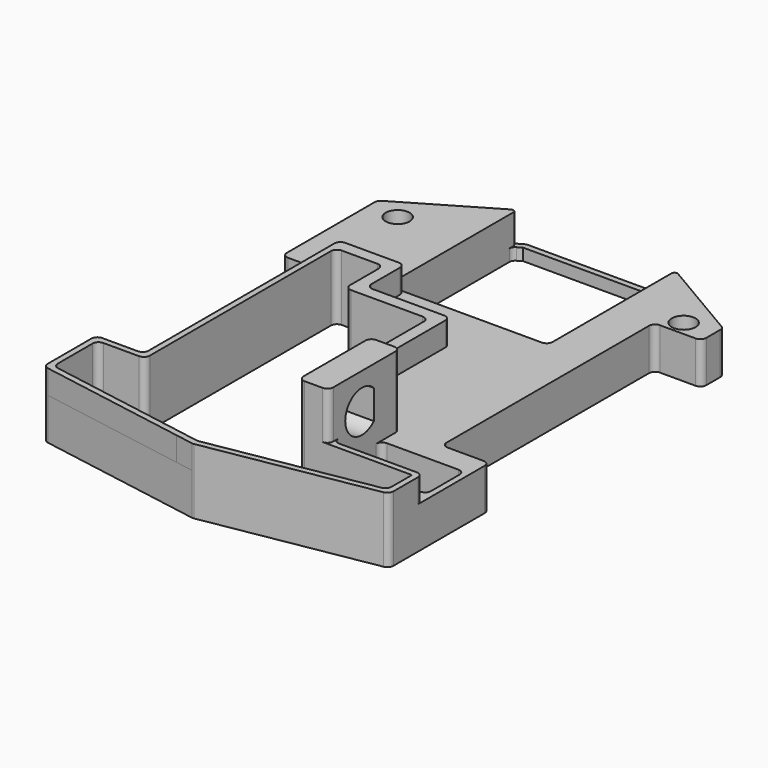
from build123d import *

# Parameters (mm, degrees)
F1_W          = 1
F1_H          = 1
F1_R          = 2
F2_DEPTH      = 7
F4_DEPTH      = 4
F6_DEPTH      = 8
F8_DEPTH      = 25
F9_W          = 1
F9_H          = 39
F10_DEPTH     = 4
F11_DEPTH     = 2
F12_T1_DEPTH  = 7
F12_T3_DEPTH  = 6.5
F12_T5_DEPTH  = 11
F12_T7_DEPTH  = 2
F12_T9_DEPTH  = 9.8597039194
F12_T11_DEPTH = 6.5
F12_T13_DEPTH = 12
F12_T15_DEPTH = 15.2116961582
F12_T17_DEPTH = 10.5
F12_T19_DEPTH = 11.8620773197
F12_T21_DEPTH = 6.5
F12_T23_DEPTH = 3.3615627907
F12_T25_DEPTH = 16
F12_T27_DEPTH = 14.5
F12_T29_DEPTH = 10.5
F12_T31_DEPTH = 24
F13_R         = 0.5


# Not quite as in the source:
# - a fillet or chamfer that OpenCascade refuses, or shapes differently, is made with other operations: its cross-section is extruded or revolved along the edge and cut away or added


with BuildPart() as f2:
    # F1 (on Top) → F2 (new body)
    with BuildSketch(Plane.XY):
        with Locations((-28.5, 11.5000484542)):
            Rectangle(F1_W, F1_H)
        Polygon((-21, 12.0000484542), (-28, 12.0000484542), (-28, 11.0000484542), (-20, 11.0000484542), (-20, 51.0000484542), (-21, 51.0000484542), align=None)
        with BuildLine():
            Line((29, 66.5), (29, 71.0000484542))
            Line((29, 71.0000484542), (14, 79.8237382314))
            Line((14, 79.8237382314), (14, 78.6635514624))
            Line((14, 78.6635514624), (14, 53.0002302017))
            Line((14, 53.0002302017), (-13, 53.0002302017))
            Line((-13, 53.0002302017), (-13, 79.2517974475))
            Line((-13, 79.2517974475), (-13, 80.4119842166))
            Line((-13, 80.4119842166), (-29, 71.0000484542))
            Line((-29, 71.0000484542), (-29, 12.0000484542))
            Line((-29, 12.0000484542), (-28, 12.0000484542))
            Line((-28, 12.0000484542), (-28, 51.0000484542))
            Line((-28, 51.0000484542), (-21, 51.0000484542))
            Line((-21, 51.0000484542), (-20, 51.0000484542))
            Line((-20, 51.0000484542), (-12, 51.0000484542))
            Line((-12, 51.0000484542), (-12, 43.0000484542))
            Line((-12, 43.0000484542), (2, 43.0000484542))
            Line((2, 43.0000484542), (2, 18))
            Line((2, 18), (9, 18))
            Line((9, 18), (14, 18))
            Line((14, 18), (28, 18))
            Line((28, 18), (28, 10.0000484542))
            Line((28, 10.0000484542), (28, 7.0000484542))
            Line((28, 7.0000484542), (28, 1.8423876859))
            Line((28, 1.8423876859), (3, -2.4679989126))
            Line((3, -2.4679989126), (3, 0))
            ThreePointArc((3, 0), (0, 3), (-3, 0))
            Line((-3, 0), (-3, -2.4679989126))
            Line((-3, -2.4679989126), (-28, 1.8423876859))
            Line((-28, 1.8423876859), (-28, 11.0000484542))
            Line((-28, 11.0000484542), (-29, 11.0000484542))
            Line((-29, 11.0000484542), (-29, 1.0000484542))
            Line((-29, 1.0000484542), (0, -4))
            Line((0, -4), (29, 1.0000484542))
            Line((29, 1.0000484542), (29, 22))
            Line((29, 22), (21, 22))
            Line((21, 22), (21, 66.5))
            Line((21, 66.5), (29, 66.5))
        make_face()
        Circle(F1_R, mode=Mode.SUBTRACT)
        with Locations((-24, 69)):
            Circle(F1_R, mode=Mode.SUBTRACT)
        with Locations((24, 69)):
            Circle(F1_R, mode=Mode.SUBTRACT)
        Polygon((9, 7.0000484542), (28, 7.0000484542), (28, 10.0000484542), (14, 10.0000484542), (14, 18), (9, 18), align=None)
    extrude(amount=F2_DEPTH)

    # F3 (on face) → F4 (join)
    with BuildSketch(Plane.XY.offset(7)):
        Polygon((4, 22), (4, 33), (4, 45.0000484542), (-10, 45.0000484542), (-10, 53.0000484542), (-21, 53.0000484542), (-21, 51.0000484542), (-21, 12.0000484542), (-28, 12.0000484542), (-29, 12.0000484542), (-29, 1.0000484542), (-3.1699085155, -3.4534587527), (0, -4), (29, 1.0000484542), (29, 8.0000484542), (14, 8.0000484542), (14, 10.0000484542), (14, 18), (14, 20), (14, 22), align=None)
        Polygon((0, -2.9852453044), (-3, -2.4679989126), (-28, 1.8423876859), (-28, 11.0000484542), (-20, 11.0000484542), (-20, 51.0000484542), (-12, 51.0000484542), (-12, 43.0000484542), (2, 43.0000484542), (2, 33), (2, 31), (2, 20), (9, 20), (9, 18), (9, 7.0000484542), (28, 7.0000484542), (28, 1.8423876859), (3, -2.4679989126), align=None, mode=Mode.SUBTRACT)
    extrude(amount=F4_DEPTH)

    # F5 (on face) → F6 (join)
    with BuildSketch(Plane.XY.offset(11)):
        Polygon((9, 20), (9, 7.0000484542), (14, 7.0000484542), (14, 8.0000484542), (14, 22), (9, 22), align=None)
    extrude(amount=F6_DEPTH)

    # F7 (on face) → F8 (cut)
    with BuildSketch(Plane.YZ.offset(29)):
        with BuildLine():
            Line((16.5000484542, 10.5505102572), (16.5000484542, 15.4494897428))
            ThreePointArc((16.5000484542, 15.4494897428), (10.5000484542, 13), (16.5000484542, 10.5505102572))
        make_face()
    extrude(amount=-F8_DEPTH, mode=Mode.SUBTRACT)

    # F9 (on face) → F10 (cut)
    with BuildSketch(Plane.XY.offset(7)):
        with Locations((-28.5, 31.5000484542)):
            Rectangle(F9_W, F9_H)
    extrude(amount=-F10_DEPTH, mode=Mode.SUBTRACT)

    # F1 (on Top) → F11 (join)
    with BuildSketch(Plane.XY):
        Polygon((14, 78.6635514624), (14, 79.8237382314), (12, 81.0002302017), (-12, 81.0002302017), (-13, 80.4119842166), (-13, 79.2517974475), (-11.7276874419, 80.0002302017), (11.7276874419, 80.0002302017), align=None)
    extrude(amount=F11_DEPTH)

    # F12: fillet of radius 1 on 48 edges, made by hand

    # F12_s2 → F12_t1 (join)
    with BuildSketch(Plane.XY):
        with BuildLine():
            ThreePointArc((-13, 54.0002302017), (-12.7071067812, 53.2931234205), (-12, 53.0002302017))
            Line((-12, 53.0002302017), (-13, 53.0002302017))
            Line((-13, 53.0002302017), (-13, 54.0002302017))
        make_face()
        with BuildLine():
            ThreePointArc((13, 53.0002302017), (13.7071067812, 53.2931234205), (14, 54.0002302017))
            Line((14, 54.0002302017), (14, 53.0002302017))
            Line((14, 53.0002302017), (13, 53.0002302017))
        make_face()
        with BuildLine():
            ThreePointArc((21, 23), (21.2928932188, 22.2928932188), (22, 22))
            Line((22, 22), (21, 22))
            Line((21, 22), (21, 23))
        make_face()
        with BuildLine():
            ThreePointArc((22, 66.5), (21.2928932188, 66.2071067812), (21, 65.5))
            Line((21, 65.5), (21, 66.5))
            Line((21, 66.5), (22, 66.5))
        make_face()
        with BuildLine():
            ThreePointArc((-22, 51.0000484542), (-21.2928932188, 50.7071552354), (-21, 50.0000484542))
            Line((-21, 50.0000484542), (-21, 51.0000484542))
            Line((-21, 51.0000484542), (-22, 51.0000484542))
        make_face()
        with BuildLine():
            ThreePointArc((14, 11.0000484542), (14.2928932188, 10.2929416731), (15, 10.0000484542))
            Line((15, 10.0000484542), (14, 10.0000484542))
            Line((14, 10.0000484542), (14, 11.0000484542))
        make_face()
        with BuildLine():
            ThreePointArc((14, 17), (14.2928932188, 17.7071067812), (15, 18))
            Line((15, 18), (14, 18))
            Line((14, 18), (14, 17))
        make_face()
        with BuildLine():
            ThreePointArc((28, 17), (27.7071067812, 17.7071067812), (27, 18))
            Line((27, 18), (28, 18))
            Line((28, 18), (28, 17))
        make_face()
        with BuildLine():
            ThreePointArc((9, 17), (8.7071067812, 17.7071067812), (8, 18))
            Line((8, 18), (9, 18))
            Line((9, 18), (9, 17))
        make_face()
        with BuildLine():
            ThreePointArc((27, 10.0000484542), (27.7071067812, 10.2929416731), (28, 11.0000484542))
            Line((28, 11.0000484542), (28, 10.0000484542))
            Line((28, 10.0000484542), (27, 10.0000484542))
        make_face()
        with BuildLine():
            ThreePointArc((-4.1699085155, -2.2662885931), (-3.3557595618, -2.0456517769), (-3, -1.2808287531))
            Line((-3, -1.2808287531), (-3, -2.4679989126))
            Line((-3, -2.4679989126), (-4.1699085155, -2.2662885931))
        make_face()
        with BuildLine():
            ThreePointArc((3, -1.2808287531), (3.3557595618, -2.0456517769), (4.1699085155, -2.2662885931))
            Line((4.1699085155, -2.2662885931), (3, -2.4679989126))
            Line((3, -2.4679989126), (3, -1.2808287531))
        make_face()
    extrude(amount=F12_T1_DEPTH)

    # F12_s4 → F12_t3 (join)
    with BuildSketch(Plane.XY.offset(4.5)):
        with BuildLine():
            ThreePointArc((-9, 45.0000484542), (-9.7071067812, 45.2929416731), (-10, 46.0000484542))
            Line((-10, 46.0000484542), (-10, 45.0000484542))
            Line((-10, 45.0000484542), (-9, 45.0000484542))
        make_face()
        with BuildLine():
            ThreePointArc((5, 22), (4.2928932188, 22.2928932188), (4, 23))
            Line((4, 23), (4, 22))
            Line((4, 22), (5, 22))
        make_face()
        with BuildLine():
            ThreePointArc((15, 8.0000484542), (14.2928932188, 8.2929416731), (14, 9.0000484542))
            Line((14, 9.0000484542), (14, 8.0000484542))
            Line((14, 8.0000484542), (15, 8.0000484542))
        make_face()
        with BuildLine():
            ThreePointArc((9, 19), (8.7071067812, 19.7071067812), (8, 20))
            Line((8, 20), (9, 20))
            Line((9, 20), (9, 19))
        make_face()
    extrude(amount=F12_T3_DEPTH)

    # F12_s6 → F12_t5 (join)
    with BuildSketch(Plane.XY):
        with BuildLine():
            ThreePointArc((-22, 12.0000484542), (-21.2928932188, 12.2929416731), (-21, 13.0000484542))
            Line((-21, 13.0000484542), (-21, 12.0000484542))
            Line((-21, 12.0000484542), (-22, 12.0000484542))
        make_face()
        with BuildLine():
            ThreePointArc((2, 42.0000484542), (1.7071067812, 42.7071552354), (1, 43.0000484542))
            Line((1, 43.0000484542), (2, 43.0000484542))
            Line((2, 43.0000484542), (2, 42.0000484542))
        make_face()
        with BuildLine():
            ThreePointArc((-12, 50.0000484542), (-12.2928932188, 50.7071552354), (-13, 51.0000484542))
            Line((-13, 51.0000484542), (-12, 51.0000484542))
            Line((-12, 51.0000484542), (-12, 50.0000484542))
        make_face()
        with BuildLine():
            ThreePointArc((-19, 51.0000484542), (-19.7071067812, 50.7071552354), (-20, 50.0000484542))
            Line((-20, 50.0000484542), (-20, 51.0000484542))
            Line((-20, 51.0000484542), (-19, 51.0000484542))
        make_face()
        with BuildLine():
            ThreePointArc((-28, 10.0000484542), (-27.7071067812, 10.7071552354), (-27, 11.0000484542))
            Line((-27, 11.0000484542), (-28, 11.0000484542))
            Line((-28, 11.0000484542), (-28, 10.0000484542))
        make_face()
        with BuildLine():
            ThreePointArc((-28, 2.6847269175), (-27.7648230238, 2.0404864793), (-27.1699085155, 1.6992670775))
            Line((-27.1699085155, 1.6992670775), (-28, 1.8423876859))
            Line((-28, 1.8423876859), (-28, 2.6847269175))
        make_face()
        with BuildLine():
            ThreePointArc((27.1699085155, 1.6992670775), (27.7648230238, 2.0404864793), (28, 2.6847269175))
            Line((28, 2.6847269175), (28, 1.8423876859))
            Line((28, 1.8423876859), (27.1699085155, 1.6992670775))
        make_face()
    extrude(amount=F12_T5_DEPTH)

    # F12_s8 → F12_t7 (join)
    with BuildSketch(Plane.XY):
        with BuildLine():
            ThreePointArc((-12.5070269726, 79.5417868517), (-12.8680515459, 79.1763307452), (-13, 78.6798566636))
            Line((-13, 78.6798566636), (-13, 79.2517974475))
            Line((-13, 79.2517974475), (-12.5070269726, 79.5417868517))
        make_face()
        with BuildLine():
            ThreePointArc((13.5070269726, 78.9535408665), (13.8680515459, 78.5880847601), (14, 78.0916106785))
            Line((14, 78.0916106785), (14, 78.6635514624))
            Line((14, 78.6635514624), (13.5070269726, 78.9535408665))
        make_face()
    extrude(amount=F12_T7_DEPTH)

    # F12_s10 → F12_t9 (cut)
    with BuildSketch(Plane.XY.offset(-1.4298519597)):
        with BuildLine():
            ThreePointArc((28.5070269726, 71.2900378584), (28.8680515459, 70.924581752), (29, 70.4281076704))
            Line((29, 70.4281076704), (29, 71.0000484542))
            Line((29, 71.0000484542), (28.5070269726, 71.2900378584))
        make_face()
        with BuildLine():
            ThreePointArc((-28.5070269726, 71.2900378584), (-28.8680515459, 70.924581752), (-29, 70.4281076704))
            Line((-29, 70.4281076704), (-29, 71.0000484542))
            Line((-29, 71.0000484542), (-28.5070269726, 71.2900378584))
        make_face()
    extrude(amount=F12_T9_DEPTH, mode=Mode.SUBTRACT)

    # F12_s12 → F12_t11 (cut)
    with BuildSketch(Plane.XY.offset(7)):
        with BuildLine():
            ThreePointArc((4, 44.0000484542), (3.7071067812, 44.7071552354), (3, 45.0000484542))
            Line((3, 45.0000484542), (4, 45.0000484542))
            Line((4, 45.0000484542), (4, 44.0000484542))
        make_face()
        with BuildLine():
            ThreePointArc((-10, 52.0000484542), (-10.2928932188, 52.7071552354), (-11, 53.0000484542))
            Line((-11, 53.0000484542), (-10, 53.0000484542))
            Line((-10, 53.0000484542), (-10, 52.0000484542))
        make_face()
        with BuildLine():
            ThreePointArc((-20, 53.0000484542), (-20.7071067812, 52.7071552354), (-21, 52.0000484542))
            Line((-21, 52.0000484542), (-21, 53.0000484542))
            Line((-21, 53.0000484542), (-20, 53.0000484542))
        make_face()
        with BuildLine():
            ThreePointArc((3, 20), (2.2928932188, 20.2928932188), (2, 21))
            Line((2, 21), (2, 20))
            Line((2, 20), (3, 20))
        make_face()
        with BuildLine():
            ThreePointArc((28, 8.0000484542), (28.7071067812, 7.7071552354), (29, 7.0000484542))
            Line((29, 7.0000484542), (29, 8.0000484542))
            Line((29, 8.0000484542), (28, 8.0000484542))
        make_face()
    extrude(amount=F12_T11_DEPTH, mode=Mode.SUBTRACT)

    # F12_s14 → F12_t13 (cut)
    with BuildSketch(Plane.XY.offset(-2.5)):
        with BuildLine():
            ThreePointArc((28, 22), (28.7071067812, 21.7071067812), (29, 21))
            Line((29, 21), (29, 22))
            Line((29, 22), (28, 22))
        make_face()
        with BuildLine():
            ThreePointArc((29, 67.5), (28.7071067812, 66.7928932188), (28, 66.5))
            Line((28, 66.5), (29, 66.5))
            Line((29, 66.5), (29, 67.5))
        make_face()
        with BuildLine():
            ThreePointArc((3, 18), (2.2928932188, 18.2928932188), (2, 19))
            Line((2, 19), (2, 18))
            Line((2, 18), (3, 18))
        make_face()
    extrude(amount=F12_T13_DEPTH, mode=Mode.SUBTRACT)

    # F12_s16 → F12_t15 (cut)
    with BuildSketch(Plane.XY.offset(-2.1058480791)):
        with BuildLine():
            ThreePointArc((29, 1.8423876859), (28.7648230238, 1.1981472477), (28.1699085155, 0.8569278458))
            Line((28.1699085155, 0.8569278458), (29, 1.0000484542))
            Line((29, 1.0000484542), (29, 1.8423876859))
        make_face()
        with BuildLine():
            ThreePointArc((-28.1699085155, 0.8569278458), (-28.7648230238, 1.1981472477), (-29, 1.8423876859))
            Line((-29, 1.8423876859), (-29, 1.0000484542))
            Line((-29, 1.0000484542), (-28.1699085155, 0.8569278458))
        make_face()
    extrude(amount=F12_T15_DEPTH, mode=Mode.SUBTRACT)

    # F12_s18 → F12_t17 (cut)
    with BuildSketch(Plane.XY.offset(3)):
        with BuildLine():
            ThreePointArc((-28, 12.0000484542), (-28.7071067812, 11.7071552354), (-29, 11.0000484542))
            Line((-29, 11.0000484542), (-29, 12.0000484542))
            Line((-29, 12.0000484542), (-28, 12.0000484542))
        make_face()
    extrude(amount=F12_T17_DEPTH, mode=Mode.SUBTRACT)

    # F12_s20 → F12_t19 (cut)
    with BuildSketch(Plane.XY.offset(-0.4310386598)):
        with BuildLine():
            ThreePointArc((-0.1699085155, -3.9707051445), (0, -3.9852453044), (0.1699085155, -3.9707051445))
            Line((0.1699085155, -3.9707051445), (0, -4))
            Line((0, -4), (-0.1699085155, -3.9707051445))
        make_face()
    extrude(amount=F12_T19_DEPTH, mode=Mode.SUBTRACT)

    # F12_s22 → F12_t21 (cut)
    with BuildSketch(Plane.XY.offset(3)):
        with BuildLine():
            ThreePointArc((-28, 51.0000484542), (-28.7071067812, 51.2929416731), (-29, 52.0000484542))
            Line((-29, 52.0000484542), (-29, 51.0000484542))
            Line((-29, 51.0000484542), (-28, 51.0000484542))
        make_face()
    extrude(amount=F12_T21_DEPTH, mode=Mode.SUBTRACT)

    # F12_s24 → F12_t23 (cut)
    with BuildSketch(Plane.XY.offset(-0.6807813954)):
        with BuildLine():
            ThreePointArc((-12.2347144144, 80.8621603897), (-11.9904323866, 80.965095526), (-11.7276874419, 81.0002302017))
            Line((-11.7276874419, 81.0002302017), (-12, 81.0002302017))
            Line((-12, 81.0002302017), (-12.2347144144, 80.8621603897))
        make_face()
        with BuildLine():
            ThreePointArc((11.7276874419, 81.0002302017), (11.9904323866, 80.965095526), (12.2347144144, 80.8621603897))
            Line((12.2347144144, 80.8621603897), (12, 81.0002302017))
            Line((12, 81.0002302017), (11.7276874419, 81.0002302017))
        make_face()
    extrude(amount=F12_T23_DEPTH, mode=Mode.SUBTRACT)

    # F12_s26 → F12_t25 (cut)
    with BuildSketch(Plane.XY.offset(-2.5)):
        with BuildLine():
            ThreePointArc((-11, 43.0000484542), (-11.7071067812, 43.2929416731), (-12, 44.0000484542))
            Line((-12, 44.0000484542), (-12, 43.0000484542))
            Line((-12, 43.0000484542), (-11, 43.0000484542))
        make_face()
        with BuildLine():
            ThreePointArc((-20, 12.0000484542), (-20.2928932188, 11.2929416731), (-21, 11.0000484542))
            Line((-21, 11.0000484542), (-20, 11.0000484542))
            Line((-20, 11.0000484542), (-20, 12.0000484542))
        make_face()
    extrude(amount=F12_T25_DEPTH, mode=Mode.SUBTRACT)

    # F12_s28 → F12_t27 (cut)
    with BuildSketch(Plane.XY.offset(7)):
        with BuildLine():
            ThreePointArc((13, 22), (13.7071067812, 21.7071067812), (14, 21))
            Line((14, 21), (14, 22))
            Line((14, 22), (13, 22))
        make_face()
    extrude(amount=F12_T27_DEPTH, mode=Mode.SUBTRACT)

    # F12_s30 → F12_t29 (cut)
    with BuildSketch(Plane.XY.offset(11)):
        with BuildLine():
            ThreePointArc((10, 22), (9.2928932188, 21.7071067812), (9, 21))
            Line((9, 21), (9, 22))
            Line((9, 22), (10, 22))
        make_face()
        with BuildLine():
            ThreePointArc((14, 8.0000484542), (13.7071067812, 7.2929416731), (13, 7.0000484542))
            Line((13, 7.0000484542), (14, 7.0000484542))
            Line((14, 7.0000484542), (14, 8.0000484542))
        make_face()
    extrude(amount=F12_T29_DEPTH, mode=Mode.SUBTRACT)

    # F12_s32 → F12_t31 (cut)
    with BuildSketch(Plane.XY.offset(-2.5)):
        with BuildLine():
            ThreePointArc((10, 7.0000484542), (9.2928932188, 7.2929416731), (9, 8.0000484542))
            Line((9, 8.0000484542), (9, 7.0000484542))
            Line((9, 7.0000484542), (10, 7.0000484542))
        make_face()
    extrude(amount=F12_T31_DEPTH, mode=Mode.SUBTRACT)

    # F13
    f13_edges = [f2.edges().sort_by_distance(p)[0] for p in [
        (-13, 80.411984, 4.5),
        (14, 79.823738, 4.5),
    ]]
    fillet(f13_edges, radius=F13_R)


solid = f2.part
